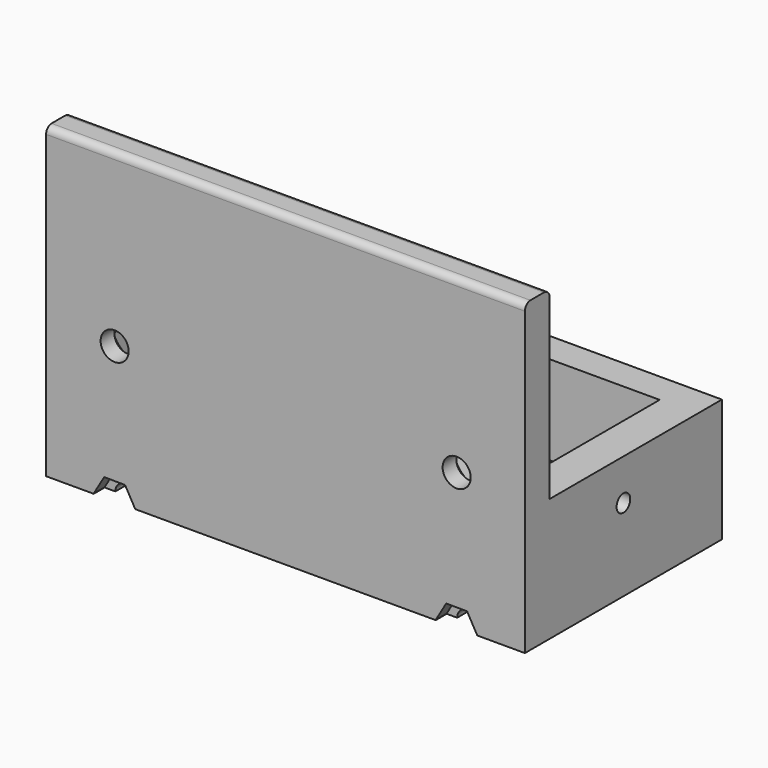
from build123d import *

# Parameters (mm, degrees)
F0_W      = 70
F0_H      = 36
F1_DEPTH  = 45
F2_W      = 59
F2_H      = 27
F3_DEPTH  = 40
F4_W      = 31.5
F4_H      = 27
F4_W_2    = 0.0242067426
F5_DEPTH  = 70.001
F6_R      = 1.25
F7_DEPTH  = 70.001
F9_DEPTH  = 2
F10_R     = 1.5
F11_DEPTH = 20
F12_R     = 2.05
F13_DEPTH = 25.4
F14_R     = 4
F14_R_2   = 2.05
F15_DEPTH = 2
F16_R     = 1


with BuildPart() as f1:
    # F0 (on Top) → F1 (new body)
    with BuildSketch(Plane.XY):
        Rectangle(F0_W, F0_H)
    extrude(amount=F1_DEPTH)

    # F2 (on face) → F3 (cut)
    with BuildSketch(Plane.XY.offset(45)):
        Rectangle(F2_W, F2_H)
    extrude(amount=-F3_DEPTH, mode=Mode.SUBTRACT)

    # F4 (on face) → F5 (cut, through all)
    with BuildSketch(Plane.YZ.offset(35)):
        with Locations((2.25, 31.5)):
            Rectangle(F4_W, F4_H)
        with Locations((18.0121033713, 31.5)):
            Rectangle(F4_W_2, F4_H)
    extrude(amount=-F5_DEPTH, mode=Mode.SUBTRACT)

    # F6 (on face) → F7 (cut, through all)
    with BuildSketch(Plane.YZ.offset(35)):
        with Locations((0, 12)):
            Circle(F6_R)
    extrude(amount=-F7_DEPTH, mode=Mode.SUBTRACT)

    # F8 (on face) → F9 (cut)
    with BuildSketch(Plane.XZ.offset(18)):
        Polygon((-28.0374098564, 0), (-21.9625901436, 0), (-23.4557936101, 2.6302886672), (-26.5057936101, 2.6524662959), (-28.05, 0.0221776287), align=None)
        Polygon((21.95, 0.0221776287), (21.9625901436, 0), (28.0374098564, 0), (26.5442063899, 2.6302886672), (23.4942063899, 2.6524662959), align=None)
    extrude(amount=-F9_DEPTH, mode=Mode.SUBTRACT)

    # F10 (on face) → F11 (cut)
    with BuildSketch(Plane.XZ.offset(16)):
        with BuildLine():
            Line((23.5, 0), (26.5, 0))
            ThreePointArc((26.5, 0), (25, 1.5), (23.5, 0))
        make_face()
        with BuildLine():
            ThreePointArc((23.5, 0), (25, -1.5), (26.5, 0))
            Line((26.5, 0), (23.5, 0))
        make_face()
        with Locations((-24.9706488103, 0)):
            Circle(F10_R)
    extrude(amount=-F11_DEPTH, mode=Mode.SUBTRACT)

    # F12 (on face) → F13 (cut)
    with BuildSketch(Plane.XZ.offset(18)):
        with Locations((-24.9807936101, 20)):
            Circle(F12_R)
        with Locations((25.0192063899, 20)):
            Circle(F12_R)
    extrude(amount=-F13_DEPTH, mode=Mode.SUBTRACT)

    # F14 (on face) → F15 (cut)
    with BuildSketch(Plane(origin=(0, -13.5, 0), x_dir=(-1, 0, 0), z_dir=(0, 1, 0))):
        with Locations((24.9807936101, 20)):
            Circle(F14_R)
        with Locations((24.9807936101, 20)):
            Circle(F14_R_2, mode=Mode.SUBTRACT)
        with Locations((-25.0192063899, 20)):
            Circle(F14_R)
        with Locations((-25.0192063899, 20)):
            Circle(F14_R_2, mode=Mode.SUBTRACT)
    extrude(amount=-F15_DEPTH, mode=Mode.SUBTRACT)

    # F16
    f16_edges = [f1.edges().sort_by_distance(p)[0] for p in [
        (0, -13.5, 45),
        (0, -18, 45),
    ]]
    fillet(f16_edges, radius=F16_R)


solid = f1.part
